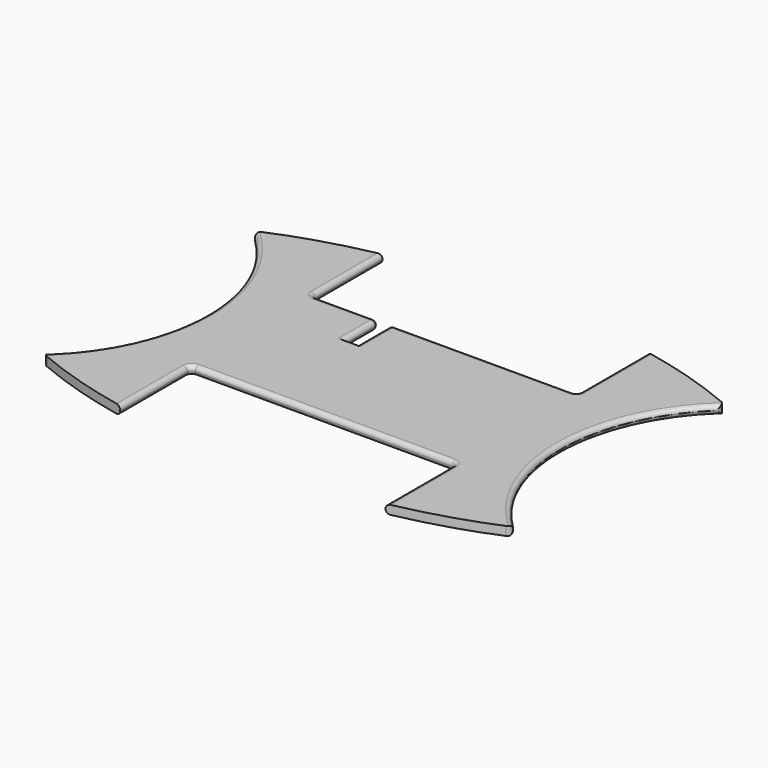
from build123d import *

# Parameters (mm, degrees)
F1_DEPTH = 2.54
F2_F1_R  = 1.27
F2_F2_R  = 1.2699


# Not quite as in the source:
# - a fillet or chamfer is up to 0.001 mm smaller than in the source, because OpenCascade refuses the exact size


with BuildPart() as f1:
    # F0 (on Top) → F1 (new body)
    with BuildSketch(Plane.XY):
        with BuildLine():
            ThreePointArc((-50.8, 0), (-55.2261567979, -20.7390131556), (-67.7333333333, -37.864084419))
            add(Edge.make_bspline(
                [(-67.7333333333, -37.864084419), (-54.52618426, -43.7705010424), (-38.1, -47.0928603931)],
                knots=[3.9826613242, 3.9826613242, 3.9826613242, 4.3279922059, 4.3279922059, 4.3279922059], degree=2, weights=[1, 0.9851303208, 1]))
            Line((-38.1, -47.0928603931), (-38.1, -21.6928603931))
            Line((-38.1, -21.6928603931), (38.1, -21.6928603931))
            Line((38.1, -21.6928603931), (38.1, -47.0928603931))
            add(Edge.make_bspline(
                [(38.1, -47.0928603931), (54.52618426, -43.7705010424), (67.7333333333, -37.864084419)],
                knots=[5.0967857549, 5.0967857549, 5.0967857549, 5.4421166366, 5.4421166366, 5.4421166366], degree=2, weights=[1, 0.9851303208, 1]))
            ThreePointArc((67.7333333333, -37.864084419), (55.2261567979, -20.7390131556), (50.8, 0))
            ThreePointArc((50.8, 0), (55.2261567979, 20.7390131556), (67.7333333333, 37.864084419))
            add(Edge.make_bspline(
                [(67.7333333333, 37.864084419), (54.52618426, 43.7705010424), (38.1, 47.0928603931)],
                knots=[0.8410686706, 0.8410686706, 0.8410686706, 1.1863995523, 1.1863995523, 1.1863995523], degree=2, weights=[1, 0.9851303208, 1]))
            Line((38.1, 47.0928603931), (38.1, 21.6928603931))
            Line((38.1, 21.6928603931), (-15.24, 21.6928603931))
            Line((-15.24, 21.6928603931), (-15.24, 8.9928603931))
            Line((-15.24, 8.9928603931), (-19.05, 8.9928603931))
            Line((-19.05, 8.9928603931), (-19.05, 21.6928603931))
            Line((-19.05, 21.6928603931), (-38.1, 21.6928603931))
            Line((-38.1, 21.6928603931), (-38.1, 47.0928603931))
            add(Edge.make_bspline(
                [(-38.1, 47.0928603931), (-54.52618426, 43.7705010424), (-67.7333333333, 37.864084419)],
                knots=[1.9551931013, 1.9551931013, 1.9551931013, 2.300523983, 2.300523983, 2.300523983], degree=2, weights=[1, 0.9851303208, 1]))
            ThreePointArc((-67.7333333333, 37.864084419), (-55.2261567979, 20.7390131556), (-50.8, 0))
        make_face()
    extrude(amount=F1_DEPTH)

    # F2: fillet of radius 1.27 on 24 edges, made by hand

    # F2_f1
    f2_f1_edges = [f1.edges().sort_by_distance(p)[0] for p in [
        (-38.1, -21.6928603931, 1.27),
        (38.1, -21.6928603931, 1.27),
        (38.1, 21.6928603931, 1.27),
        (-38.1, 21.6928603931, 1.27),
    ]]
    fillet(f2_f1_edges, radius=F2_F1_R)

    # F2_f2 (radius 1.27 in the source; OpenCascade refuses exactly that, so slightly less here)
    f2_f2_edges = [f1.edges().sort_by_distance(p)[0] for p in [
        (67.7333333333, -37.864084419, 1.27),
        (50.8, 0, 2.54),
        (67.7333333333, 37.864084419, 1.27),
        (50.8, 0, 0),
        (0, -21.6928603931, 0),
        (0, -21.6928603931, 2.54),
        (-67.7333333333, 37.864084419, 1.27),
        (-50.8, 0, 2.54),
        (-67.7333333333, -37.864084419, 1.27),
        (-50.8, 0, 0),
        (-15.24, 21.6928603931, 1.27),
        (10.795, 21.6928603931, 0),
        (10.795, 21.6928603931, 2.54),
        (-19.05, 21.6928603931, 1.27),
        (-27.94, 21.6928603931, 0),
        (-27.94, 21.6928603931, 2.54),
        (-15.24, 15.3428603931, 2.54),
        (-19.05, 15.3428603931, 2.54),
        (-15.24, 15.3428603931, 0),
        (-19.05, 15.3428603931, 0),
        (-37.7280256121, 22.064834781, 2.54),
        (-37.7280256121, 22.064834781, 0),
        (37.7280256121, 22.064834781, 2.54),
        (37.7280256121, 22.064834781, 0),
        (-37.7280256121, -22.064834781, 2.54),
        (37.7280256121, -22.064834781, 2.54),
        (-37.7280256121, -22.064834781, 0),
        (37.7280256121, -22.064834781, 0),
    ]]
    fillet(f2_f2_edges, radius=F2_F2_R)


solid = f1.part
